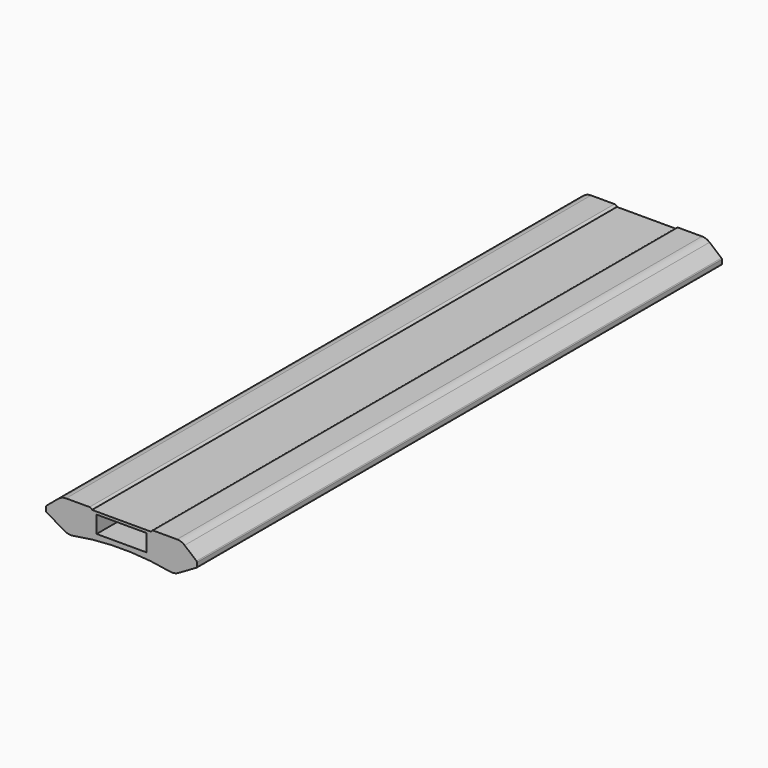
from build123d import *

# Parameters (mm, degrees)
F1_DEPTH    = 250
F2_W        = 38
F2_H        = 13
F3_DEPTH    = 500.001
F4_T1_DEPTH = 509.3674969976
F5_R        = 9
F6_R        = 1


# Not quite as in the source:
# - a fillet or chamfer that OpenCascade refuses, or shapes differently, is made with other operations: its cross-section is extruded or revolved along the edge and cut away or added


with BuildPart() as f1:
    # F0 (on Front) → F1 (new body, symmetric)
    with BuildSketch(Plane.XZ):
        with BuildLine():
            Line((22.5, 22.7), (0, 22.7))
            Line((0, 22.7), (-22.5, 22.7))
            Line((-22.5, 22.7), (-22.5, 24))
            Line((-22.5, 24), (-45.5824640741, 24))
            Line((-45.5824640741, 24), (-57.5, 14))
            Line((-57.5, 14), (-57.5, 10))
            Line((-57.5, 10), (-40.1794919243, 0))
            ThreePointArc((-40.1794919243, 0), (0, 4.0775448584), (40.1794919243, 0))
            Line((40.1794919243, 0), (57.5, 10))
            Line((57.5, 10), (57.5, 14))
            Line((57.5, 14), (45.5824640741, 24))
            Line((45.5824640741, 24), (22.5, 24))
            Line((22.5, 24), (22.5, 22.7))
        make_face()
    extrude(amount=F1_DEPTH, both=True)

    # F2 (on face) → F3 (cut, through all)
    with BuildSketch(Plane.XZ.offset(250)):
        with Locations((0, 14.2)):
            Rectangle(F2_W, F2_H)
    extrude(amount=-F3_DEPTH, mode=Mode.SUBTRACT)

    # F4: fillet of radius 2 on 2 edges, made by hand

    # F4_s2 → F4_t1 (cut)
    with BuildSketch(Plane.XZ.offset(-254.6837484988)):
        with BuildLine():
            ThreePointArc((-24.3734993995, 24), (-23.2333239744, 23.6431676725), (-22.5, 22.7))
            Line((-22.5, 22.7), (-22.5, 24))
            Line((-22.5, 24), (-24.3734993995, 24))
        make_face()
        with BuildLine():
            ThreePointArc((24.3734993995, 24), (23.2333239744, 23.6431676725), (22.5, 22.7))
            Line((22.5, 22.7), (22.5, 24))
            Line((22.5, 24), (24.3734993995, 24))
        make_face()
    extrude(amount=F4_T1_DEPTH, mode=Mode.SUBTRACT)

    # F5
    f5_edges = [f1.edges().sort_by_distance(p)[0] for p in [
        (-45.582464, 0, 24),
        (45.582464, 0, 24),
        (-40.179492, 0, 0),
        (40.179492, 0, 0),
    ]]
    fillet(f5_edges, radius=F5_R)

    # F6
    f6_edges = [f1.edges().sort_by_distance(p)[0] for p in [
        (42.306732, 0, 24),
        (57.5, 0, 14),
        (57.5, 0, 10),
        (-57.5, 0, 10),
        (-57.5, 0, 14),
    ]]
    fillet(f6_edges, radius=F6_R)


solid = f1.part
